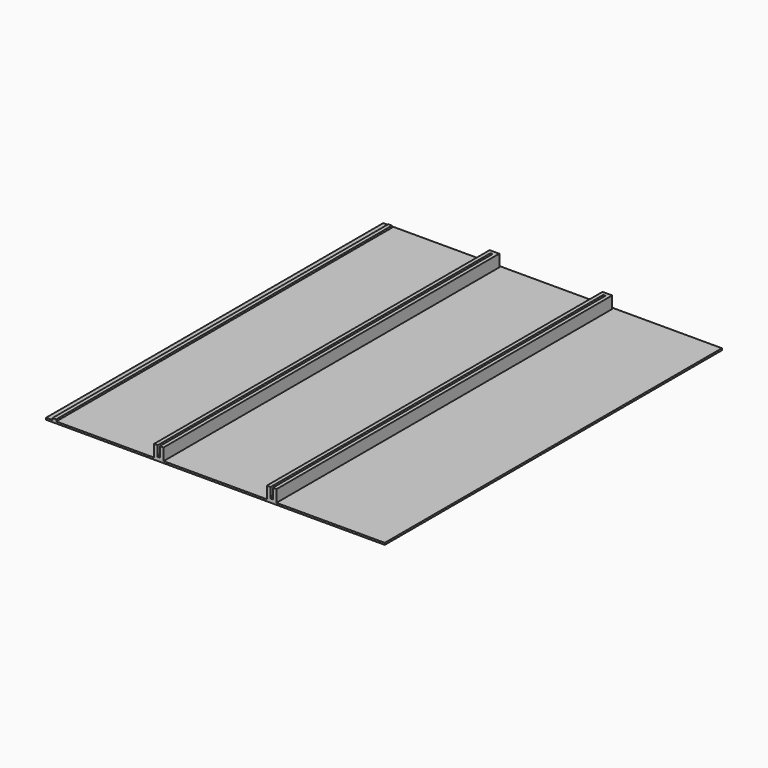
from build123d import *

# Parameters (mm, degrees)
F0_W     = 5.2
F0_H     = 226.71
F1_DEPTH = 2
F3_DEPTH = 4.5
F4_W     = 1.2
F4_H     = 2.1
F5_DEPTH = 25
F6_W     = 183
F6_H     = 227.71
F7_DEPTH = 1
F8_W     = 2
F8_H     = 226.71
F9_DEPTH = 1
F10_SIZE = 1


# Not quite as in the source:
# - a feature names something its author has since deleted; it is built from what else it names


with BuildPart() as f1:
    # F0 (on Top) → F1 (new body)
    with BuildSketch(Plane.XY):
        with Locations((2.6, 113.355)):
            Rectangle(F0_W, F0_H)
    extrude(amount=F1_DEPTH)

    # F2 (on face) → F3 (join)
    with BuildSketch(Plane.XY.offset(2)):
        Polygon((0, 226.71), (0, 0), (2, 0), (2, 224.71), (3.2, 224.71), (3.2, 0), (5.2, 0), (5.2, 226.71), align=None)
    extrude(amount=F3_DEPTH)


with BuildPart() as f1b:
    # F0 (on Top) → F1, piece 2 (new body)
    with BuildSketch(Plane.XY):
        with Locations((63.6, 113.355)):
            Rectangle(F0_W, F0_H)
    extrude(amount=F1_DEPTH)

    # F2 (on face) → F3, piece 2 (join)
    with BuildSketch(Plane.XY.offset(2)):
        Polygon((61, 226.71), (61, 0), (63, 0), (63, 224.71), (64.2, 224.71), (64.2, 0), (66.2, 0), (66.2, 226.71), align=None)
    extrude(amount=F3_DEPTH)


with BuildPart() as f5_tool:
    # F4 (on face) → F5 (new body)
    with BuildSketch(Plane.XY.offset(2)):
        with Locations((2.6, 2.95)):
            Rectangle(F4_W, F4_H)
        with Locations((63.6, 2.95)):
            Rectangle(F4_W, F4_H)
    extrude(amount=-F5_DEPTH)


with BuildPart() as f1_1:
    add(f1.part)

    # F5: cut by f5_tool
    add(f5_tool.part, mode=Mode.SUBTRACT)



with BuildPart() as f1b_1:
    add(f1b.part)

    # F5: cut by f5_tool
    add(f5_tool.part, mode=Mode.SUBTRACT)


with BuildPart() as f1_2:
    add(f1_1.part)

    add(f1b_1.part)  # F7 merges F1b
    # F6 (on Top) → F7 (join)
    with BuildSketch(Plane.XY):
        with Locations((33.2, 113.855)):
            Rectangle(F6_W, F6_H)
    extrude(amount=-F7_DEPTH)

    # F8 (on face) → F9 (join)
    with BuildSketch(Plane.XY):
        with Locations((-53.8, 113.355)):
            Rectangle(F8_W, F8_H)
    extrude(amount=F9_DEPTH)

    # F10
    f10_edges = [f1_2.edges().sort_by_distance(p)[0] for p in [
        (2.6, 0, 2),
        (63.6, 0, 2),
    ]]
    chamfer(f10_edges, length=F10_SIZE)


solid = f1_2.part
